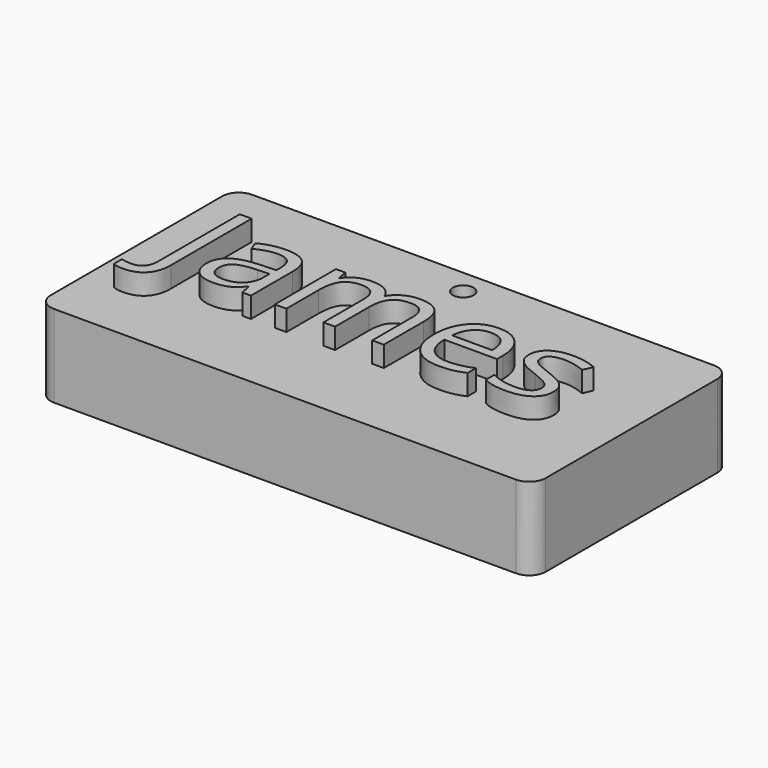
from build123d import *

# Parameters (mm, degrees)
F0_W         = 76.2
F0_H         = 38.1
F1_DEPTH     = 12.7
F2_TEXT_SIZE = 21.9842042627
F3_DEPTH     = 3.175
F4_R         = 1.5875
F5_DEPTH     = 25.4
F6_R         = 2.54


# Not quite as in the source:
# - Text() gives the source's letters only with a copy of the font that has no kerning and outlines rounded to 1/6400 em; it was checked with that copy


with BuildPart() as f1:
    # F0 (on Top) → F1 (new body)
    with BuildSketch(Plane.XY):
        Rectangle(F0_W, F0_H)
    extrude(amount=F1_DEPTH)

    # F2 (on face) → F3 (join)
    with BuildSketch(Plane.XY.offset(12.7)):
        with Locations((-31.75, -6.3036270691)):
            Text('James', F2_TEXT_SIZE, font='Open Sans', text_align=(TextAlign.LEFT, TextAlign.BOTTOM))
    extrude(amount=F3_DEPTH)

    # F4 (on face) → F5 (cut)
    with BuildSketch(Plane.XY.offset(12.7)):
        with Locations((0, 15.24)):
            Circle(F4_R)
    extrude(amount=-F5_DEPTH, mode=Mode.SUBTRACT)

    # F6
    f6_edges = [f1.edges().sort_by_distance(p)[0] for p in [
        (38.1, 19.05, 6.35),
        (-38.1, 19.05, 6.35),
        (-38.1, -19.05, 6.35),
        (38.1, -19.05, 6.35),
    ]]
    fillet(f6_edges, radius=F6_R)


solid = f1.part
